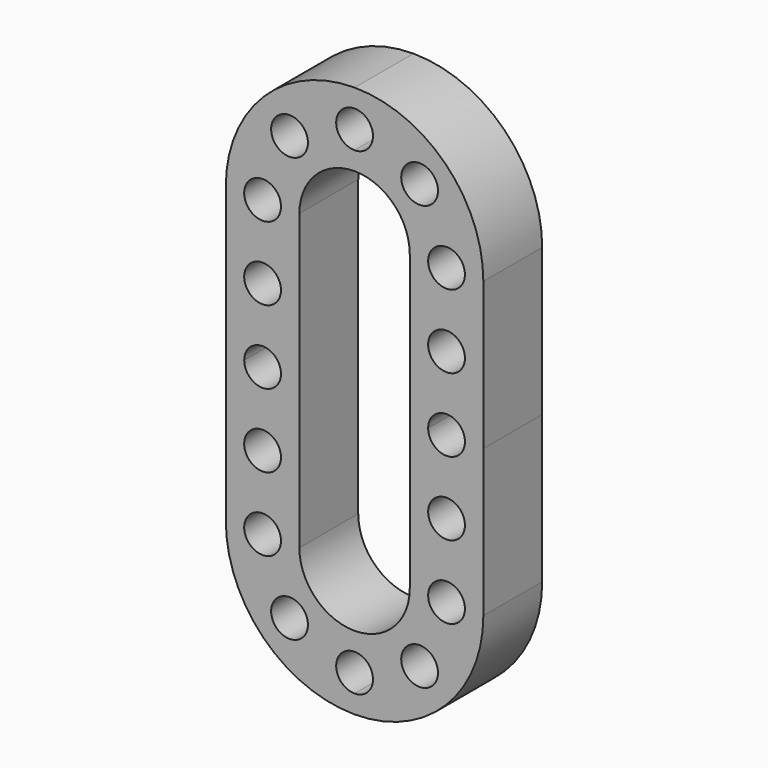
from build123d import *
from build123d import SkipClean  # not in build123d's __all__

# Parameters (mm, degrees)
F0_R     = 5
F1_DEPTH = 20


with BuildPart() as f1:
    # F0 (on Front) → F1 (new body)
    with BuildSketch(Plane.XZ):
        with BuildLine():
            ThreePointArc((-15, 40), (-10.6066017178, 50.6066017178), (0, 55))
            Line((0, 55), (0, 60))
            ThreePointArc((0, 60), (-5, 65), (0, 70))
            Line((0, 70), (0, 75))
            ThreePointArc((0, 75), (-24.7487373415, 64.7487373415), (-35, 40))
            Line((-35, 40), (-35, 0))
            Line((-35, 0), (-30, 0))
            ThreePointArc((-30, 0), (-25, 5), (-20, 0))
            Line((-20, 0), (-15, 0))
            Line((-15, 0), (-15, 40))
        make_face()
        with Locations((-25, 20)):
            Circle(F0_R, mode=Mode.SUBTRACT)
        with Locations((-25, 40)):
            Circle(F0_R, mode=Mode.SUBTRACT)
        with Locations((-17.6776695297, 57.6776695297)):
            Circle(F0_R, mode=Mode.SUBTRACT)
    extrude(amount=F1_DEPTH)

    # F2: F1 across plane


with BuildPart() as f1_1:
    add(f1.part, clean=False)
    with SkipClean():  # cleaning this boolean's faces spoils the solid; the shape is the same uncleaned
        add(f1.part.mirror(Plane.YZ), clean=False)

    # F3: F1 across plane


with BuildPart() as f1_2:
    add(f1_1.part, clean=False)
    add(f1_1.part.mirror(Plane.XY), clean=False)


solid = f1_2.part
